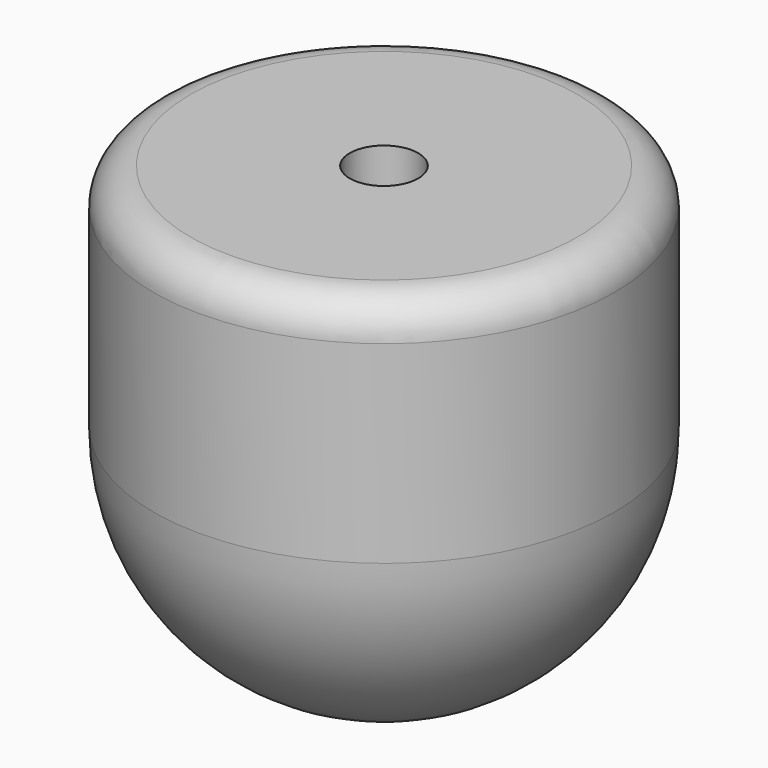
from build123d import *

# Parameters (mm, degrees)
F3_R = 5.08
F5_R = 5.08


# Not quite as in the source:
# - a feature names something its author has since deleted; it is built from what else it names


with BuildPart() as f1:
    # F0 (on Front) → F1 (revolve)
    with BuildSketch(Plane.XZ):
        with BuildLine():
            Line((0, -5.842), (0, 0))
            Line((0, 0), (0, 3.81))
            Line((0, 3.81), (0, 16.51))
            Line((0, 16.51), (0, 26.035))
            Line((0, 26.035), (-4.7244, 26.035))
            Line((-4.7244, 26.035), (-4.7244, 35.56))
            Line((-4.7244, 35.56), (-7.2644, 35.56))
            Line((-7.2644, 35.56), (-31.75, 35.56))
            Line((-31.75, 35.56), (-31.75, 3.81))
            ThreePointArc((-31.75, 3.81), (-24.2400753332, -16.6956394155), (-5.2629922621, -27.5007555394))
            Line((-5.2629922621, -27.5007555394), (-1.6002, -27.8064487898))
            Line((-1.6002, -27.8064487898), (-1.6002, -5.842))
            Line((-1.6002, -5.842), (0, -5.842))
        make_face()
    revolve(axis=Axis((0, 0, 3.81), (0, 0, 1)))

    # F5
    f5_edges = [f1.edges().sort_by_distance(p)[0] for p in [
        (31.75, 0, 35.56),
    ]]
    fillet(f5_edges, radius=F5_R)


with BuildPart() as f2:
    # F0 (on Front) → F2 (revolve)
    with BuildSketch(Plane.XZ):
        with BuildLine():
            Line((0, -5.842), (0, 0))
            Line((0, 0), (0, 3.81))
            Line((0, 3.81), (0, 16.51))
            Line((0, 16.51), (0, 26.035))
            Line((0, 26.035), (-4.7244, 26.035))
            Line((-4.7244, 26.035), (-4.7244, 35.56))
            Line((-4.7244, 35.56), (-7.2644, 35.56))
            Line((-7.2644, 35.56), (-31.75, 35.56))
            Line((-31.75, 35.56), (-31.75, 3.81))
            ThreePointArc((-31.75, 3.81), (-24.2400753332, -16.6956394155), (-5.2629922621, -27.5007555394))
            Line((-5.2629922621, -27.5007555394), (-1.6002, -27.8064487898))
            Line((-1.6002, -27.8064487898), (-1.6002, -5.842))
            Line((-1.6002, -5.842), (0, -5.842))
        make_face()
    revolve(axis=Axis((0, 0, 3.81), (0, 0, 1)))

    # F3
    f3_edges = [f2.edges().sort_by_distance(p)[0] for p in [
        (31.75, 0, 35.56),
    ]]
    fillet(f3_edges, radius=F3_R)


solid = f1.part
